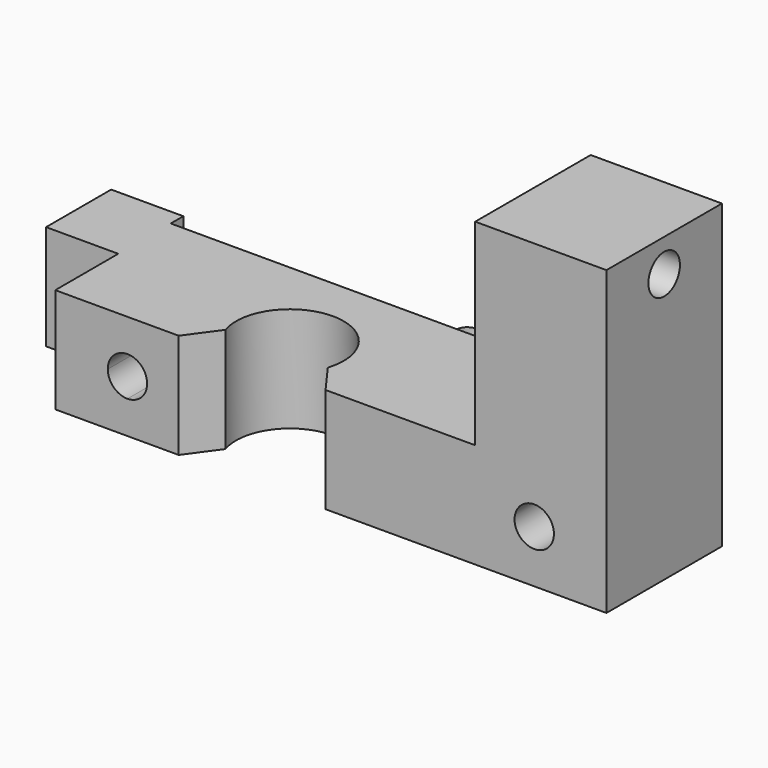
from build123d import *

# Parameters (mm, degrees)
F1_W         = 42
F1_H         = 11
F2_DEPTH     = 8
F3_R         = 4.1
F4_DEPTH     = 25
F5_T1_DEPTH  = 27.0282480506
F7_DEPTH     = 25
F8_TEXT_SIZE = 11.1111111111
F9_DEPTH     = 1
F10_W        = 10
F10_H        = 11
F11_DEPTH    = 15
F12_R        = 1.5
F13_DEPTH    = 25
F14_W        = 6.2
F14_H        = 8
F15_DEPTH    = 5.5


# Not quite as in the source:
# - a fillet or chamfer that OpenCascade refuses, or shapes differently, is made with other operations: its cross-section is extruded or revolved along the edge and cut away or added
# - Text() gives the source's letters only with a copy of the font that has no kerning and outlines rounded to 1/6400 em; it was checked with that copy


with BuildPart() as f2:
    # F1 (on Top) → F2 (new body)
    with BuildSketch(Plane.XY):
        with Locations((21, 5.5)):
            Rectangle(F1_W, F1_H)
    extrude(amount=F2_DEPTH)

    # F3 (on face) → F4 (cut)
    with BuildSketch(Plane.XY.offset(8)):
        with Locations((15, 3.6)):
            Circle(F3_R)
    extrude(amount=-F4_DEPTH, mode=Mode.SUBTRACT)

    # F5: chamfer of 7 on 2 edges, made by hand

    # F5_s2 → F5_t1 (cut)
    with BuildSketch(Plane.XY.offset(-9.5141240253)):
        with BuildLine():
            Line((20.7610452751, -0.2264961011), (18.73515334, 2.5608842714))
            Line((18.73515334, 2.5608842714), (18.6019903715, 2.6041002851))
            ThreePointArc((18.6019903715, 2.6041002851), (18.0707550937, 1.0995874031), (16.895141727, 0.1229268293))
            Line((16.895141727, 0.1229268293), (16.962141687, -0.14))
            ThreePointArc((16.962141687, -0.14), (18.861593481, -0.14), (20.7610452751, -0.3664961011))
            Line((20.7610452751, -0.3664961011), (20.7610452751, -0.2264961011))
        make_face()
        with BuildLine():
            Line((11.26484666, 2.5608842714), (9.2389547249, -0.2264961011))
            Line((9.2389547249, -0.2264961011), (9.2389547249, -0.3664961011))
            ThreePointArc((9.2389547249, -0.3664961011), (11.138406519, -0.14), (13.037858313, -0.14))
            Line((13.037858313, -0.14), (13.104858273, 0.1229268293))
            ThreePointArc((13.104858273, 0.1229268293), (11.9292449063, 1.0995874031), (11.3980096285, 2.6041002851))
            Line((11.3980096285, 2.6041002851), (11.26484666, 2.5608842714))
        make_face()
    extrude(amount=F5_T1_DEPTH, mode=Mode.SUBTRACT)

    # F6 (on face) → F7 (cut)
    with BuildSketch(Plane(origin=(0, 11, 0), x_dir=(-1, 0, 0), z_dir=(0, 1, 0))):
        with BuildLine():
            Line((-5.5, 4), (-4, 4))
            ThreePointArc((-4, 4), (-4.4393398282, 5.0606601718), (-5.5, 5.5))
            Line((-5.5, 5.5), (-5.5, 4))
        make_face()
        with BuildLine():
            ThreePointArc((-5.5, 2.5), (-4.4393398282, 2.9393398282), (-4, 4))
            Line((-4, 4), (-5.5, 4))
            Line((-5.5, 4), (-5.5, 2.5))
        make_face()
        with BuildLine():
            Line((-5.5, 4), (-5.5, 5.5))
            ThreePointArc((-5.5, 5.5), (-7, 4), (-5.5, 2.5))
            Line((-5.5, 2.5), (-5.5, 4))
        make_face()
        with BuildLine():
            ThreePointArc((-38, 4), (-36.5, 2.5), (-35, 4))
            ThreePointArc((-35, 4), (-36.5, 5.5), (-38, 4))
        make_face()
    extrude(amount=-F7_DEPTH, mode=Mode.SUBTRACT)

    # F8 (on face) → F9 (join)
    with BuildSketch(Plane(origin=(0, 11, 0), x_dir=(-1, 0, 0), z_dir=(0, 1, 0))):
        with Locations((-26.7275573479, 0)):
            Text('R', F8_TEXT_SIZE, font='Open Sans', font_style=FontStyle.BOLD, text_align=(TextAlign.LEFT, TextAlign.BOTTOM))
    extrude(amount=F9_DEPTH)

    # F10 (on face) → F11 (join)
    with BuildSketch(Plane.XY.offset(8)):
        with Locations((37, 5.5)):
            Rectangle(F10_W, F10_H)
    extrude(amount=F11_DEPTH)

    # F12 (on face) → F13 (cut)
    with BuildSketch(Plane.YZ.offset(42)):
        with Locations((5.5, 20.5)):
            Circle(F12_R)
    extrude(amount=-F13_DEPTH, mode=Mode.SUBTRACT)

    # F14 (on face) → F15 (join)
    with BuildSketch(Plane(origin=(0, 0, 0), x_dir=(0, -1, 0), z_dir=(-1, 0, 0))):
        with Locations((-9.1, 4)):
            Rectangle(F14_W, F14_H)
    extrude(amount=F15_DEPTH)


solid = f2.part
